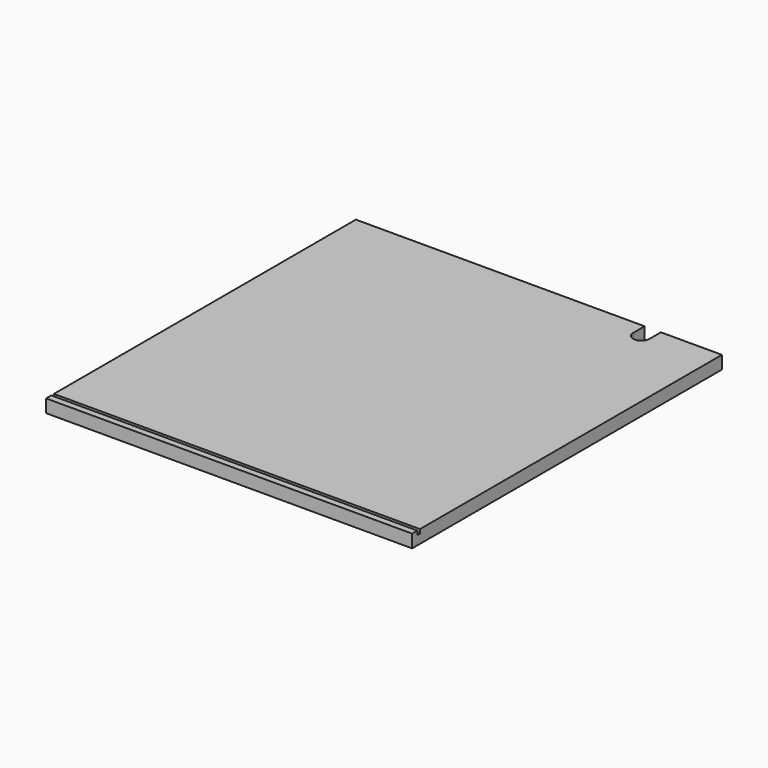
from build123d import *

# Parameters (mm, degrees)
F0_W     = 450
F0_H     = 476
F1_DEPTH = 8
F3_DEPTH = 16.001
F4_W     = 4
F4_H     = 5
F5_DEPTH = 450.001


# Not quite as in the source:
# - a feature names something its author has since deleted; it is built from what else it names


with BuildPart() as f1:
    # F0 (on Top) → F1 (new body, symmetric)
    with BuildSketch(Plane.XY):
        Rectangle(F0_W, F0_H)
    extrude(amount=F1_DEPTH, both=True)

    # F2 (on face) → F3 (cut, through all)
    with BuildSketch(Plane.XY.offset(8)):
        with BuildLine():
            ThreePointArc((149.9904602378, 220.9366969629), (140.0025066822, 230.4999996858), (130.0097599498, 220.9417054897))
            ThreePointArc((130.0097599498, 220.9417054897), (139.5607987599, 210.5096495421), (149.9904602378, 220.0633030371))
            Line((149.9904602378, 220.0633030371), (149.9904602378, 220.9366969629))
        make_face()
        with BuildLine():
            Line((149.9904602378, 220.9366969629), (149.9904602378, 220.0633030371))
            ThreePointArc((149.9904602378, 220.0633030371), (149.997614775, 220.2815994251), (150, 220.5))
            ThreePointArc((150, 220.5), (149.997614775, 220.7184005749), (149.9904602378, 220.9366969629))
        make_face()
        with BuildLine():
            Line((130.0097599498, 238), (130.0097599498, 220.9417054897))
            ThreePointArc((130.0097599498, 220.9417054897), (140.0025066822, 230.4999996858), (149.9904602378, 220.9366969629))
            Line((149.9904602378, 220.9366969629), (149.9904602378, 238))
            Line((149.9904602378, 238), (130.0097599498, 238))
        make_face()
    extrude(amount=-F3_DEPTH, mode=Mode.SUBTRACT)

    # F4 (on face) → F5 (cut, through all)
    with BuildSketch(Plane.YZ.offset(225)):
        with Locations((-228, 5.5)):
            Rectangle(F4_W, F4_H)
    extrude(amount=-F5_DEPTH, mode=Mode.SUBTRACT)


solid = f1.part
